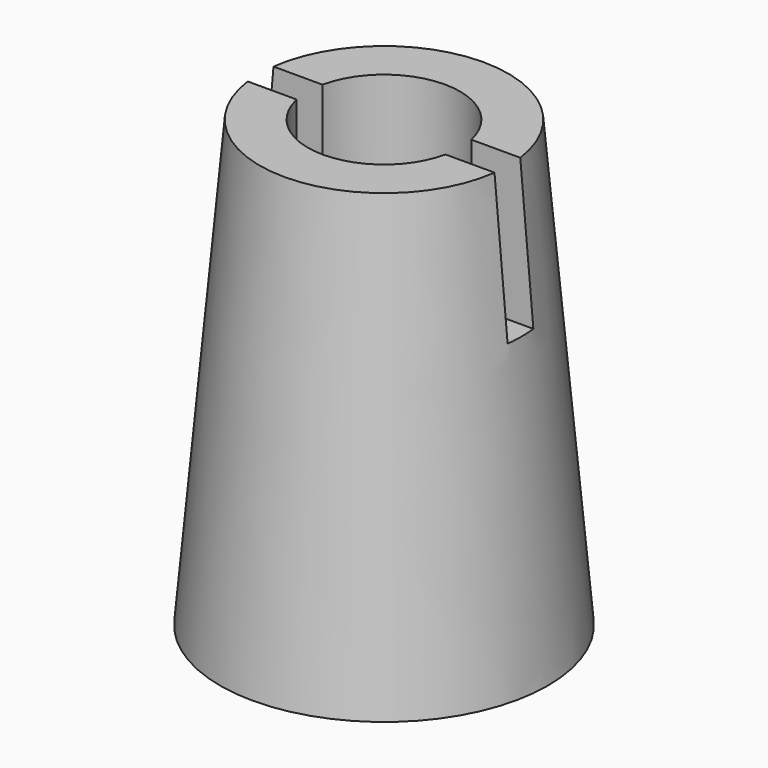
from build123d import *

# Parameters (mm, degrees)
F2_R     = 10.625
F0_R     = 14
F4_R     = 3.75
F5_DEPTH = 61.90218
F7_DEPTH = 12.5
F9_D     = 13
F9_DEPTH = 8.5
F9_TIP   = 3.9055940237


with BuildPart() as f3:
    # F2 (on offset) → F3 section 0
    with BuildSketch(Plane.XY.offset(38)):
        Circle(F2_R)
    # F0 (on Top) → F3 section 1
    with BuildSketch(Plane.XY):
        Circle(F0_R)
    loft()

    # F4 (on Top) → F5 (cut)
    with BuildSketch(Plane.XY):
        Circle(F4_R)
    extrude(amount=F5_DEPTH, mode=Mode.SUBTRACT)

    # F6 (on face) → F7 (cut)
    with BuildSketch(Plane.XY.offset(38)):
        with BuildLine():
            Line((-10.5356537529, 1.375), (-16.0871957117, 1.375))
            Line((-16.0871957117, 1.375), (-16.0871957117, 0))
            Line((-16.0871957117, 0), (-10.625, 0))
            ThreePointArc((-10.625, 0), (-10.60263991, 0.6889498806), (-10.5356537529, 1.375))
        make_face()
        with BuildLine():
            Line((-3.4888214342, 1.375), (-10.5356537529, 1.375))
            ThreePointArc((-10.5356537529, 1.375), (-10.60263991, 0.6889498806), (-10.625, 0))
            Line((-10.625, 0), (-3.75, 0))
            ThreePointArc((-3.75, 0), (-3.6841267879, 0.6997926913), (-3.4888214342, 1.375))
        make_face()
        with BuildLine():
            Line((-10.625, 0), (-16.0871957117, 0))
            Line((-16.0871957117, 0), (-16.0871957117, -1.375))
            Line((-16.0871957117, -1.375), (-10.5356537529, -1.375))
            ThreePointArc((-10.5356537529, -1.375), (-10.60263991, -0.6889498806), (-10.625, 0))
        make_face()
        with BuildLine():
            ThreePointArc((10.625, 0), (10.60263991, 0.6889498806), (10.5356537529, 1.375))
            Line((10.5356537529, 1.375), (3.4888214342, 1.375))
            ThreePointArc((3.4888214342, 1.375), (3.6841267879, 0.6997926913), (3.75, 0))
            Line((3.75, 0), (10.625, 0))
        make_face()
        with BuildLine():
            Line((16.6521480927, 1.375), (10.5356537529, 1.375))
            ThreePointArc((10.5356537529, 1.375), (10.60263991, 0.6889498806), (10.625, 0))
            Line((10.625, 0), (16.6521480927, 0))
            Line((16.6521480927, 0), (16.6521480927, 1.375))
        make_face()
        with BuildLine():
            Line((-3.75, 0), (-10.625, 0))
            ThreePointArc((-10.625, 0), (-10.60263991, -0.6889498806), (-10.5356537529, -1.375))
            Line((-10.5356537529, -1.375), (-3.4888214342, -1.375))
            ThreePointArc((-3.4888214342, -1.375), (-3.6841267879, -0.6997926913), (-3.75, 0))
        make_face()
        with BuildLine():
            ThreePointArc((10.5356537529, -1.375), (10.60263991, -0.6889498806), (10.625, 0))
            Line((10.625, 0), (3.75, 0))
            ThreePointArc((3.75, 0), (3.6841267879, -0.6997926913), (3.4888214342, -1.375))
            Line((3.4888214342, -1.375), (10.5356537529, -1.375))
        make_face()
        with BuildLine():
            Line((16.6521480927, 0), (10.625, 0))
            ThreePointArc((10.625, 0), (10.60263991, -0.6889498806), (10.5356537529, -1.375))
            Line((10.5356537529, -1.375), (16.6521480927, -1.375))
            Line((16.6521480927, -1.375), (16.6521480927, 0))
        make_face()
    extrude(amount=-F7_DEPTH, mode=Mode.SUBTRACT)

    # F9
    with Locations(Plane.XY.offset(38)):
        with Locations((0, 0)):
            Hole(F9_D / 2, depth=F9_DEPTH)
            with Locations((0, 0, -(F9_DEPTH + F9_TIP / 2))):  # 118° drill point
                Cone(0, F9_D / 2, F9_TIP, mode=Mode.SUBTRACT)


solid = f3.part
